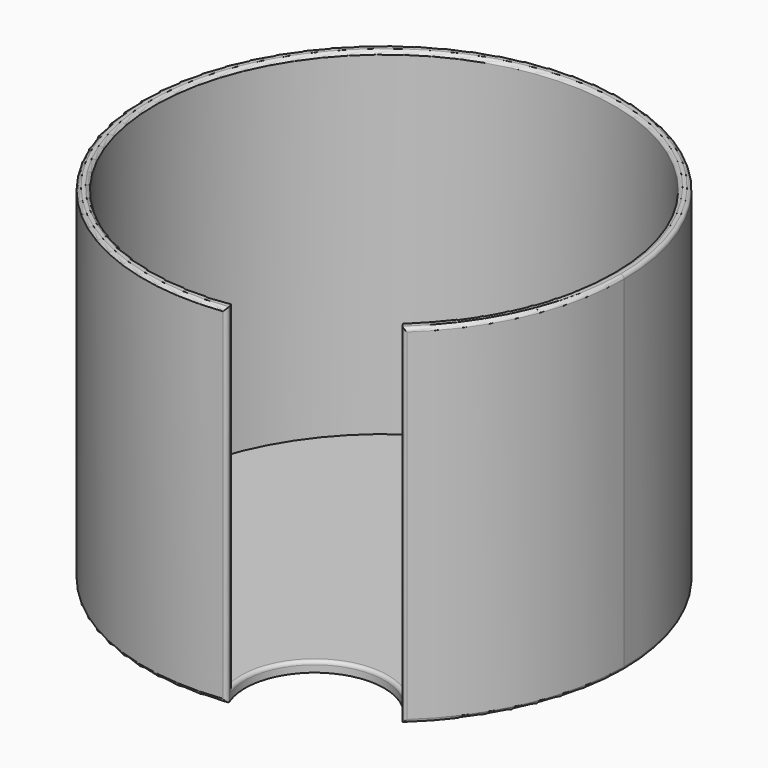
from build123d import *

# Parameters (mm, degrees)
F1_DEPTH = 50
F2_T     = -1.5
F3_R     = 0.5


with BuildPart() as f1:
    # F0 (on Top) → F1 (new body)
    with BuildSketch(Plane.XY):
        with BuildLine():
            ThreePointArc((-30.9694676058, 4.9068101727), (-22.4931361106, 16.5301319793), (-19.493863568, 30.599750654))
            ThreePointArc((-19.493863568, 30.599750654), (-80.0641317689, 53.196013972), (-49.0933485496, -3.5504316669))
            ThreePointArc((-49.0933485496, -3.5504316669), (-44.2600289976, 9.7401297248), (-30.9694676058, 4.9068101727))
        make_face()
    extrude(amount=F1_DEPTH)

    # F2
    f2_openings = [f1.faces().sort_by_distance(p)[0] for p in [
        (-54.609526, 31.919117, 50),
        (-44.260029, 9.74013, 25),
    ]]
    offset(amount=F2_T, openings=f2_openings)

    # F3
    f3_edges = [f1.edges().sort_by_distance(p)[0] for p in [
        (-68.582606, 61.863445, 50),
        (-67.948313, 60.504154, 50),
        (-49.634541, -2.111047, 25.75),
        (-30.969468, 4.90681, 25),
        (-31.724949, 6.2462, 25.75),
        (-44.260029, 9.74013, 1.5),
        (-68.582606, 61.863445, 0),
        (-49.093349, -3.550432, 25),
    ]]
    fillet(f3_edges, radius=F3_R)


solid = f1.part
